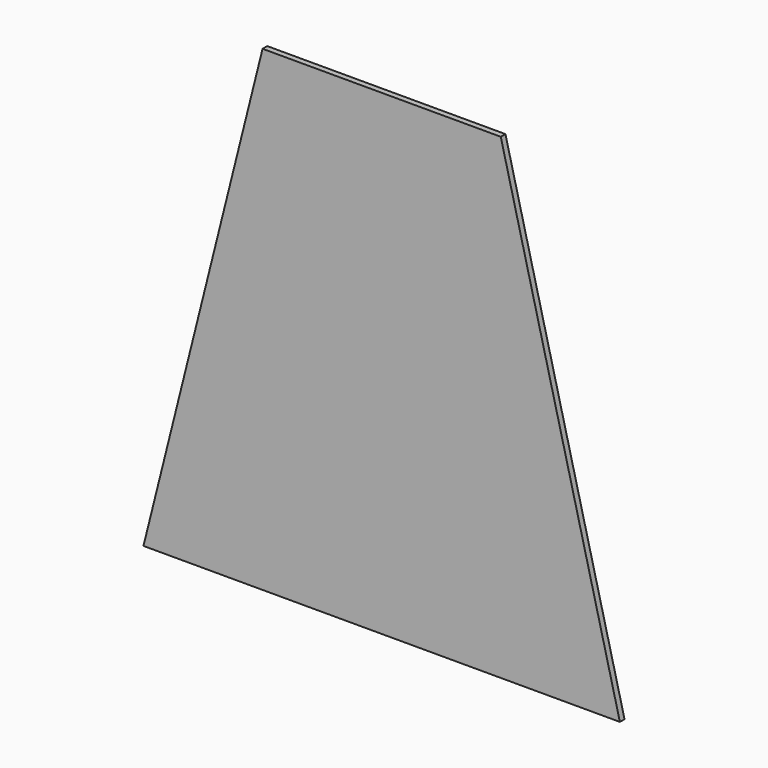
from build123d import *

# Parameters (mm, degrees)
F1_DEPTH = 1.5875


# Not quite as in the source:
# - a length typed as a fraction of an inch, garbled in the dataset ("3 / 203.2 mm" for 3/8 in), is restored


with BuildPart() as f1:
    # F0 (on Front) → F1 (new body, symmetric)
    with BuildSketch(Plane.XZ):
        Polygon((-64.77, 259.08), (-129.54, 0), (0, 0), (0, 259.08), align=None)
        Polygon((0, 259.08), (0, 0), (129.54, 0), (64.77, 259.08), align=None)
    extrude(amount=F1_DEPTH, both=True)


solid = f1.part
